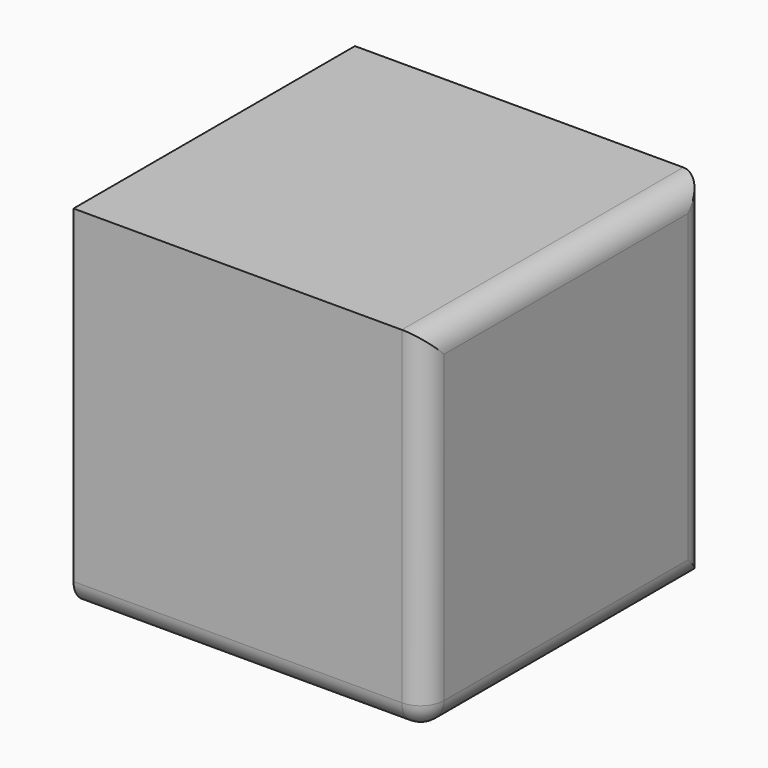
from build123d import *

# Parameters (mm, degrees)
F0_W         = 76.2
F0_H         = 76.2
F1_DEPTH     = 76.2
F2_T         = -2.54
F3_T1_DEPTH  = 83.82
F3_T3_DEPTH  = 83.82
F3_T5_DEPTH  = 83.82
F3_T7_DEPTH  = 101.6
F3_T9_DEPTH  = 101.6
F3_S13_W     = 5.08
F3_S13_H     = 5.08
F3_T14_DEPTH = 5.08


# Not quite as in the source:
# - a fillet or chamfer that OpenCascade refuses, or shapes differently, is made with other operations: its cross-section is extruded or revolved along the edge and cut away or added


with BuildPart() as f1:
    # F0 (on Front) → F1 (new body)
    with BuildSketch(Plane.XZ):
        with Locations((-1.2479908764, -6.1416627283)):
            Rectangle(F0_W, F0_H)
    extrude(amount=F1_DEPTH)

    # F2
    f2_openings = [f1.faces().sort_by_distance(p)[0] for p in [
        (-1.247991, 0, -6.141663),
    ]]
    offset(amount=F2_T, openings=f2_openings)

    # F3: fillet of radius 5.08 on 5 edges, made by hand

    # F3_s2 → F3_t1 (cut)
    with BuildSketch(Plane.XY.offset(-39.1616627283)):
        with BuildLine():
            ThreePointArc((36.8520091236, -71.12), (35.364111572, -74.7121024484), (31.7720091236, -76.2))
            Line((31.7720091236, -76.2), (36.8520091236, -76.2))
            Line((36.8520091236, -76.2), (36.8520091236, -71.12))
        make_face()
    extrude(amount=F3_T1_DEPTH, mode=Mode.SUBTRACT)

    # F3_s4 → F3_t3 (cut)
    with BuildSketch(Plane.YZ.offset(-52.0479908764)):
        with BuildLine():
            ThreePointArc((-71.12, -44.2416627283), (-74.7121024484, -42.7537651767), (-76.2, -39.1616627283))
            Line((-76.2, -39.1616627283), (-76.2, -44.2416627283))
            Line((-76.2, -44.2416627283), (-71.12, -44.2416627283))
        make_face()
    extrude(amount=F3_T3_DEPTH, mode=Mode.SUBTRACT)

    # F3_s6 → F3_t5 (cut)
    with BuildSketch(Plane.XZ.offset(-12.7)):
        with BuildLine():
            ThreePointArc((31.7720091236, -44.2416627283), (35.364111572, -42.7537651767), (36.8520091236, -39.1616627283))
            Line((36.8520091236, -39.1616627283), (36.8520091236, -44.2416627283))
            Line((36.8520091236, -44.2416627283), (31.7720091236, -44.2416627283))
        make_face()
    extrude(amount=F3_T5_DEPTH, mode=Mode.SUBTRACT)

    # F3_s8 → F3_t7 (cut)
    with BuildSketch(Plane.XY.offset(-56.9416627283)):
        with BuildLine():
            ThreePointArc((36.8520091236, -5.08), (35.364111572, -1.4878975516), (31.7720091236, 0))
            Line((31.7720091236, 0), (36.8520091236, 0))
            Line((36.8520091236, 0), (36.8520091236, -5.08))
        make_face()
    extrude(amount=F3_T7_DEPTH, mode=Mode.SUBTRACT)

    # F3_s10 → F3_t9 (cut)
    with BuildSketch(Plane.XZ.offset(-12.7)):
        with BuildLine():
            ThreePointArc((31.7720091236, 31.9583372717), (35.364111572, 30.4704397201), (36.8520091236, 26.8783372717))
            Line((36.8520091236, 26.8783372717), (36.8520091236, 31.9583372717))
            Line((36.8520091236, 31.9583372717), (31.7720091236, 31.9583372717))
        make_face()
    extrude(amount=F3_T9_DEPTH, mode=Mode.SUBTRACT)


with BuildPart() as f3_tool12:
    # F3_s13 → F3_t14 (new body)
    with BuildSketch(Plane.XY.offset(-39.1616627283)):
        with Locations((34.3120091236, -73.66)):
            Rectangle(F3_S13_W, F3_S13_H)
    extrude(amount=-F3_T14_DEPTH)

    # F3_s15 → F3_t16 (revolve, cut)
    with BuildSketch(Plane(origin=(31.7720091236, -71.12, -39.1616627283), x_dir=(-0.7071067812, 0.7071067812, 0), z_dir=(-0.7071067812, -0.7071067812, 0))):
        with BuildLine():
            ThreePointArc((0, -5.08), (5.08, 0), (0, 5.08))
            Line((0, 5.08), (0, -5.08))
        make_face()
    revolve(axis=Axis((31.7720091236, -71.12, -39.1616627283), (0, 0, -1)), mode=Mode.SUBTRACT)


with BuildPart() as f1_1:
    add(f1.part)

    # F3_t11: cut F3_tool12
    add(f3_tool12.part, mode=Mode.SUBTRACT)


solid = f1_1.part
